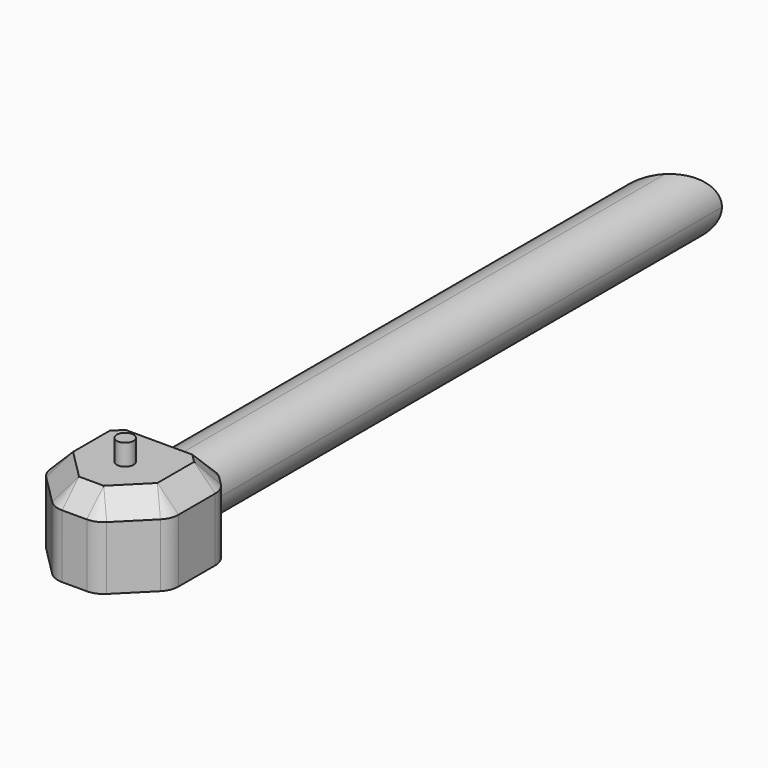
from build123d import *

# Parameters (mm, degrees)
F1_DEPTH  = 15
F2_R      = 7.49999
F3_W      = 30
F3_H      = 30
F4_DEPTH  = 20
F5_SIZE   = 10
F6_SIZE   = 5
F7_R      = 5
F8_SIZE   = 4.99999
F9_R      = 2
F10_DEPTH = 5


# Not quite as in the source:
# - a fillet or chamfer is up to 0.001 mm smaller than in the source, because OpenCascade refuses the exact size


with BuildPart() as f1:
    # F0 (on Top) → F1 (new body)
    with BuildSketch(Plane.XY):
        Polygon((0, 150), (0, 12.5), (15, 12.5), (15, 165), align=None)
    extrude(amount=F1_DEPTH)

    # F2 (radius 7.5 in the source; OpenCascade refuses exactly that, so slightly less here)
    f2_edges = [f1.edges().sort_by_distance(p)[0] for p in [
        (15, 88.75, 15),
        (0, 81.25, 15),
        (0, 81.25, 0),
        (15, 88.75, 0),
    ]]
    fillet(f2_edges, radius=F2_R)

    # F3 (on Top) → F4 (join)
    with BuildSketch(Plane.XY):
        with Locations((7.5, -2.5)):
            Rectangle(F3_W, F3_H)
    extrude(amount=F4_DEPTH)

    # F5
    f5_edges = [f1.edges().sort_by_distance(p)[0] for p in [
        (-7.5, -17.5, 10),
        (22.5, -17.5, 10),
    ]]
    chamfer(f5_edges, length=F5_SIZE)

    # F6
    f6_edges = [f1.edges().sort_by_distance(p)[0] for p in [
        (22.5, 12.5, 10),
        (-7.5, 12.5, 10),
    ]]
    chamfer(f6_edges, length=F6_SIZE)

    # F7
    f7_edges = [f1.edges().sort_by_distance(p)[0] for p in [
        (12.5, -17.5, 10),
        (2.5, -17.5, 10),
        (-7.5, -7.5, 10),
        (22.5, -7.5, 10),
        (22.5, 7.5, 10),
        (17.5, 12.5, 10),
        (-2.5, 12.5, 10),
        (-7.5, 7.5, 10),
    ]]
    fillet(f7_edges, radius=F7_R)

    # F8 (size 5 in the source; OpenCascade refuses exactly that, so slightly less here)
    f8_edges = [f1.edges().sort_by_distance(p)[0] for p in [
        (22.5, 0, 20),
        (22.119398, -7.342349, 20),
        (22.119398, 7.342349, 20),
        (17.5, -12.5, 20),
        (20, 10, 20),
        (12.342349, -17.119398, 20),
        (17.342349, 12.119398, 20),
        (7.5, -17.5, 20),
        (7.5, 12.5, 20),
        (2.657651, -17.119398, 20),
        (-2.342349, 12.119398, 20),
        (-2.5, -12.5, 20),
        (-5, 10, 20),
        (-7.119398, -7.342349, 20),
        (-7.119398, 7.342349, 20),
        (-7.5, 0, 20),
    ]]
    chamfer(f8_edges, length=F8_SIZE)

    # F9 (on face) → F10 (join)
    with BuildSketch(Plane.XY.offset(20)):
        with Locations((7.5, -2.5)):
            Circle(F9_R)
    extrude(amount=F10_DEPTH)


solid = f1.part
